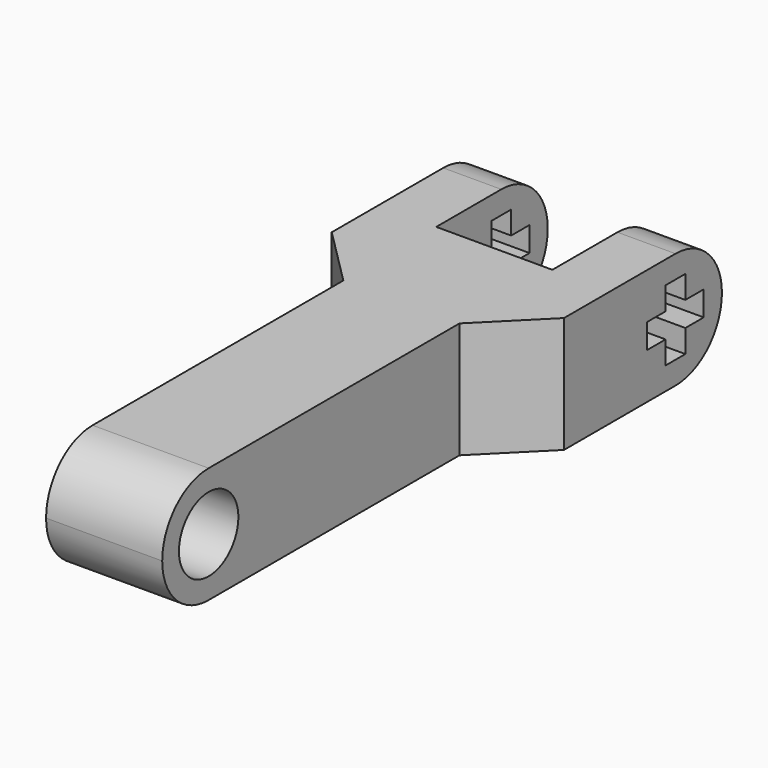
from build123d import *

# Parameters (mm, degrees)
F0_W     = 7.9375
F0_H     = 25.4
F1_DEPTH = 7.9375
F2_R     = 3.96874
F3_W     = 1.6891
F3_H     = 1.56845
F3_W_2   = 1.56845
F3_H_2   = 1.6891
F3_R     = 2.54
F4_DEPTH = 15.875


# Not quite as in the source:
# - a fillet or chamfer is up to 0.001 mm smaller than in the source, because OpenCascade refuses the exact size


with BuildPart() as f1:
    # F0 (on Top) → F1 (new body)
    with BuildSketch(Plane.XY):
        Polygon((-3.96875, 3.96875), (0, 0), (7.9375, 0), (11.90625, 3.96875), (11.90625, 17.4625), (7.9375, 17.4625), (7.9375, 7.9375), (0, 7.9375), (0, 17.4625), (-3.96875, 17.4625), align=None)
        with Locations((3.96875, -12.7)):
            Rectangle(F0_W, F0_H)
    extrude(amount=F1_DEPTH)

    # F2 (radius 3.96875 in the source; OpenCascade refuses exactly that, so slightly less here)
    f2_edges = [f1.edges().sort_by_distance(p)[0] for p in [
        (3.96875, -25.4, 7.9375),
        (3.96875, -25.4, 0),
        (9.921875, 17.4625, 7.9375),
        (9.921875, 17.4625, 0),
        (-1.984375, 17.4625, 7.9375),
        (-1.984375, 17.4625, 0),
    ]]
    fillet(f2_edges, radius=F2_R)

    # F3 (on face) → F4 (cut, through all)
    with BuildSketch(Plane.YZ.offset(11.90625)):
        with Locations((13.49375, 5.597525)):
            Rectangle(F3_W, F3_H)
        with Locations((15.122525, 3.96875)):
            Rectangle(F3_W_2, F3_H_2)
        with Locations((13.49375, 3.96875)):
            Rectangle(F3_W, F3_H_2)
        with Locations((11.864975, 3.96875)):
            Rectangle(F3_W_2, F3_H_2)
        with Locations((13.49375, 2.339975)):
            Rectangle(F3_W, F3_H)
        with Locations((-21.43125, 3.96875)):
            Circle(F3_R)
    extrude(amount=-F4_DEPTH, mode=Mode.SUBTRACT)


solid = f1.part
